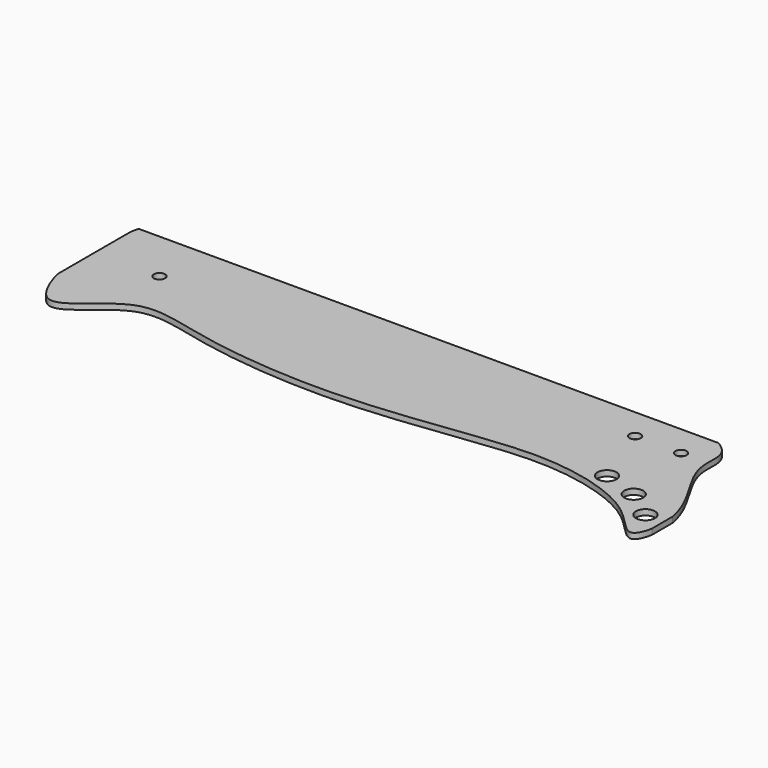
from build123d import *

# Parameters (mm, degrees)
F0_W     = 1433.8989723474
F0_H     = 383.8273435831
F1_DEPTH = 12.7
F3_DEPTH = 12.701
F4_R     = 12.7
F5_DEPTH = 25.4
F6_R     = 21.59
F7_DEPTH = 12.7010001


with BuildPart() as f1:
    # F0 (on Top) → F1 (new body)
    with BuildSketch(Plane.XY):
        with Locations((736.9271283969, -72.5835487247)):
            Rectangle(F0_W, F0_H)
    extrude(amount=F1_DEPTH)

    # F2 (on face) → F3 (cut, through all)
    with BuildSketch(Plane.XY.offset(12.7)):
        with BuildLine():
            add(Edge.make_bspline(
                [(23.8233897985, 119.3301230669), (21.6565458101, 112.3890118703), (20.6756031882, 104.8809228493), (19.9776422232, 96.7474654317)],
                knots=[0.0325304406, 0.0325304406, 0.0325304406, 0.0325304406, 0.044354018, 0.044354018, 0.044354018, 0.044354018], degree=3))
            Line((23.8233897985, 119.3301230669), (19.9776422232, 119.3301230669))
            Line((19.9776422232, 119.3301230669), (19.9776422232, 96.7474654317))
        make_face()
        with BuildLine():
            Line((1453.8766145706, 119.3301230669), (1340.4833078385, 119.3301230669))
            add(Edge.make_bspline(
                [(1453.8766145706, -152.7797728777), (1444.8861721142, -100.0066257216), (1386.4830680217, -21.8819630361), (1367.5935234806, 47.5566795571), (1379.6596673526, 97.7256977198), (1340.4833078384, 119.3301230669)],
                knots=[0.7069290309, 0.7069290309, 0.7069290309, 0.7069290309, 0.76224488, 0.7996241078, 0.8396558499, 0.8396558499, 0.8396558499, 0.8396558499], degree=3))
            Line((1453.8766145706, -152.7797728777), (1453.8766145706, 119.3301230669))
        make_face()
        with BuildLine():
            add(Edge.make_bspline(
                [(1453.8766145707, -211.3673318743), (1456.9659425303, -194.3252836531), (1457.3377944757, -173.0966101579), (1453.8766145706, -152.7797728777)],
                knots=[0.6856332931, 0.6856332931, 0.6856332931, 0.6856332931, 0.7069290309, 0.7069290309, 0.7069290309, 0.7069290309], degree=3))
            Line((1453.8766145706, -152.7797728777), (1453.8766145706, -211.3673318743))
        make_face()
        with BuildLine():
            Line((1453.8766145706, -264.4972205162), (1453.8766145706, -211.3673318743))
            add(Edge.make_bspline(
                [(19.9776422232, -103.9730086923), (24.3756687382, -128.300707788), (53.9404162103, -207.3482977869), (118.18563376, -180.1775685975), (208.841378416, -83.5676493307), (375.0429052781, -141.2900206769), (687.6951980634, -171.8723737776), (994.404795869, -125.2501516946), (1179.2519608483, -111.4952047309), (1368.4012079058, -167.4873842097), (1432.3799684146, -267.8037059643), (1450.5861550866, -229.5189072101), (1453.8766145707, -211.3673318743)],
                knots=[0.1521586148, 0.1521586148, 0.1521586148, 0.1521586148, 0.1959270808, 0.2281980685, 0.2773216753, 0.3343115246, 0.4155599093, 0.4955701148, 0.5575423121, 0.6208385182, 0.6629510906, 0.6856332931, 0.6856332931, 0.6856332931, 0.6856332931], degree=3))
            Line((19.9776422232, -103.9730086922), (19.9776422232, -264.4972205162))
            Line((19.9776422232, -264.4972205162), (1453.8766145706, -264.4972205162))
        make_face()
    extrude(amount=-F3_DEPTH, mode=Mode.SUBTRACT)

    # F4 (on face) → F5 (cut)
    with BuildSketch(Plane.XY.offset(12.7)):
        with Locations((166.6177362204, 0)):
            Circle(F4_R)
        with BuildLine():
            Line((1221.5536024094, 47.6566180587), (1196.1536024094, 47.6566180587))
            ThreePointArc((1196.1536024094, 47.6566180587), (1208.8536024094, 34.9566180587), (1221.5536024094, 47.6566180587))
        make_face()
        with BuildLine():
            ThreePointArc((1221.5536024094, 47.6566180587), (1208.8536024094, 60.3566180587), (1196.1536024094, 47.6566180587))
            Line((1196.1536024094, 47.6566180587), (1221.5536024094, 47.6566180587))
        make_face()
        with BuildLine():
            ThreePointArc((1325.9092952728, 47.6566180587), (1313.2092952728, 60.3566180587), (1300.5092952728, 47.6566180587))
            ThreePointArc((1300.5092952728, 47.6566180587), (1313.2092952728, 34.9566180587), (1325.9092952728, 47.6566180587))
        make_face()
    extrude(amount=-F5_DEPTH, mode=Mode.SUBTRACT)

    # F6 (on face) → F7 (cut, through all)
    with BuildSketch(Plane.XY.offset(12.7)):
        with Locations((1411.8106365204, -176.8049150705)):
            Circle(F6_R)
        with Locations((1346.2386131287, -128.1287372112)):
            Circle(F6_R)
        with Locations((1264.9775743484, -102.3826450109)):
            Circle(F6_R)
    extrude(amount=-F7_DEPTH, mode=Mode.SUBTRACT)


solid = f1.part
